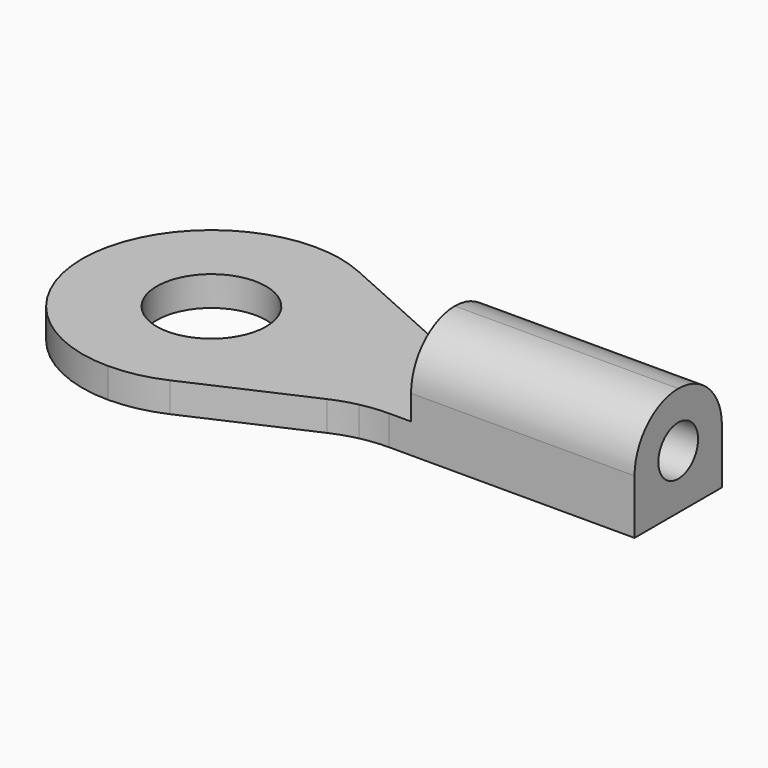
from build123d import *

# Parameters (mm, degrees)
F0_W     = 4.5
F0_H     = 2.2
F0_R     = 1.1
F1_DEPTH = 0.6
F2_W     = 4.5
F2_H     = 2.2
F3_DEPTH = 1.6
F4_R     = 1.09999
F5_R     = 0.5
F6_DEPTH = 10


# Not quite as in the source:
# - a fillet or chamfer is up to 0.001 mm smaller than in the source, because OpenCascade refuses the exact size


with BuildPart() as f1:
    # F0 (on Top) → F1 (new body)
    with BuildSketch(Plane.XY):
        with Locations((9.75, 2.6)):
            Rectangle(F0_W, F0_H)
        with BuildLine():
            Line((7.0565025569, 1.5), (7.5, 1.5))
            Line((7.5, 1.5), (7.5, 3.7))
            Line((7.5, 3.7), (7.0565025569, 3.7))
            ThreePointArc((7.0565025569, 3.7), (6.7766250144, 3.7151076306), (6.5, 3.7602549529))
            ThreePointArc((6.5, 3.7602549529), (6.2418088438, 3.8309365837), (5.9922537502, 3.9277912239))
            Line((5.9922537502, 3.9277912239), (3.6642488067, 4.9722087761))
            ThreePointArc((3.6642488067, 4.9722087761), (3.1441769851, 5.1424144841), (2.6, 5.2))
            ThreePointArc((2.6, 5.2), (0.7615223689, 4.4384776311), (0, 2.6))
            ThreePointArc((0, 2.6), (0.7615223689, 0.7615223689), (2.6, 0))
            ThreePointArc((2.6, 0), (3.1441769851, 0.0575855159), (3.6642488067, 0.2277912239))
            Line((3.6642488067, 0.2277912239), (5.9922537502, 1.2722087761))
            ThreePointArc((5.9922537502, 1.2722087761), (6.2418088438, 1.3690634163), (6.5, 1.4397450471))
            ThreePointArc((6.5, 1.4397450471), (6.7766250144, 1.4848923694), (7.0565025569, 1.5))
        make_face()
        with Locations((2.6, 2.6)):
            Circle(F0_R, mode=Mode.SUBTRACT)
    extrude(amount=F1_DEPTH)

    # F2 (on face) → F3 (join)
    with BuildSketch(Plane.XY.offset(0.6)):
        with Locations((9.75, 2.6)):
            Rectangle(F2_W, F2_H)
    extrude(amount=F3_DEPTH)

    # F4 (radius 1.1 in the source; OpenCascade refuses exactly that, so slightly less here)
    f4_edges = [f1.edges().sort_by_distance(p)[0] for p in [
        (9.75, 1.5, 2.2),
        (9.75, 3.7, 2.2),
    ]]
    fillet(f4_edges, radius=F4_R)

    # F5 (on face) → F6 (cut)
    with BuildSketch(Plane.YZ.offset(12)):
        with Locations((2.6, 1.1)):
            Circle(F5_R)
    extrude(amount=-F6_DEPTH, mode=Mode.SUBTRACT)


solid = f1.part
